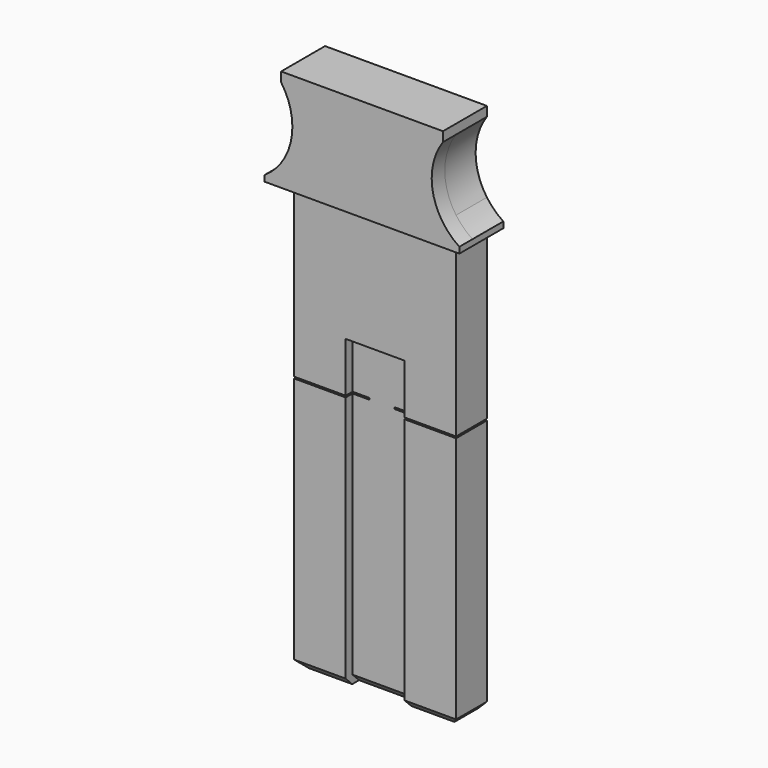
from build123d import *

# Parameters (mm, degrees)
F1_DEPTH = 4.7
F3_DEPTH = 1.05
F6_DEPTH = 2
F7_SIZE  = 1


with BuildPart() as f1:
    # F0 (on Front) → F1 (new body)
    with BuildSketch(Plane.XZ):
        with BuildLine():
            Line((0, 31.2), (0, 0))
            Line((0, 0), (19.75, 0))
            Line((19.75, 0), (19.75, 31.2))
            Line((19.75, 31.2), (11.425, 31.2))
            Line((11.425, 31.2), (11.425, 31.4))
            Line((11.425, 31.4), (19.75, 31.4))
            Line((19.75, 31.4), (19.75, 52.5))
            Line((19.75, 52.5), (19.75, 55.1716775767))
            ThreePointArc((19.75, 55.1716775767), (18.375, 59.5), (19.75, 63.8283224233))
            Line((19.75, 63.8283224233), (19.75, 65))
            Line((19.75, 65), (0, 65))
            Line((0, 65), (0, 63.8283224233))
            ThreePointArc((0, 63.8283224233), (1.0229892277, 61.7707377656), (1.375, 59.5))
            ThreePointArc((1.375, 59.5), (1.0229892277, 57.2292622344), (0, 55.1716775767))
            Line((0, 55.1716775767), (0, 52.5))
            Line((0, 52.5), (0, 31.4))
            Line((0, 31.4), (8.325, 31.4))
            Line((8.325, 31.4), (8.325, 31.2))
            Line((8.325, 31.2), (0, 31.2))
        make_face()
        with BuildLine():
            Line((-2, 52.5), (0, 52.5))
            Line((0, 52.5), (0, 55.1716775767))
            ThreePointArc((0, 55.1716775767), (-0.9094386331, 54.1103878035), (-2, 53.2362650918))
            Line((-2, 53.2362650918), (-2, 52.5))
        make_face()
        with BuildLine():
            Line((19.75, 55.1716775767), (19.75, 52.5))
            Line((19.75, 52.5), (21.75, 52.5))
            Line((21.75, 52.5), (21.75, 53.2362650918))
            ThreePointArc((21.75, 53.2362650918), (20.6594386331, 54.1103878035), (19.75, 55.1716775767))
        make_face()
    extrude(amount=F1_DEPTH)

    # F2 (on face) → F3 (cut)
    with BuildSketch(Plane.XZ.offset(4.7)):
        Polygon((13.475, 37.5), (6.275, 37.5), (6.275, 2.2), (6.275, 0), (13.475, 0), (13.475, 2.2), align=None)
    extrude(amount=-F3_DEPTH, mode=Mode.SUBTRACT)

    # F5 (on face) → F6 (join)
    with BuildSketch(Plane.XZ.offset(4.7)):
        with BuildLine():
            Line((-2, 52.5), (0, 52.5))
            Line((0, 52.5), (19.75, 52.5))
            Line((19.75, 52.5), (21.75, 52.5))
            Line((21.75, 52.5), (21.75, 53.2362650918))
            ThreePointArc((21.75, 53.2362650918), (18.5052276407, 58.1084342015), (19.75, 63.8283224233))
            Line((19.75, 63.8283224233), (19.75, 65))
            Line((19.75, 65), (0, 65))
            Line((0, 65), (0, 63.8283224233))
            ThreePointArc((0, 63.8283224233), (1.2447723593, 58.1084342015), (-2, 53.2362650918))
            Line((-2, 53.2362650918), (-2, 52.5))
        make_face()
    extrude(amount=F6_DEPTH)

    # F7
    f7_edges = [f1.edges().sort_by_distance(p)[0] for p in [
        (0, -2.35, 0),
        (19.75, -2.35, 0),
        (3.1375, -4.7, 0),
        (16.6125, -4.7, 0),
        (9.875, -3.65, 0),
    ]]
    chamfer(f7_edges, length=F7_SIZE)


solid = f1.part
